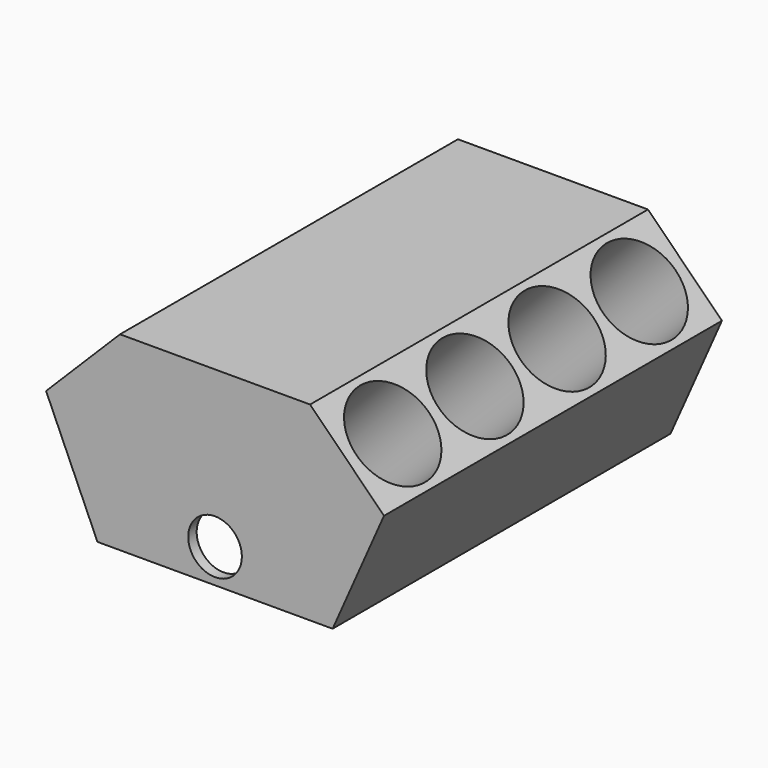
from build123d import *

# Parameters (mm, degrees)
F1_DEPTH  = 100
F2_R      = 21.59
F4_DEPTH  = 52
F3_R      = 21.59
F5_DEPTH  = 52
F6_DEPTH  = 2.5
F7_DEPTH  = 95
F8_DEPTH  = 2.5
F3_R_2    = 24
F9_DEPTH  = 51
F10_START = 43.5
F10_DEPTH = 5
F11_START = 43.5
F11_DEPTH = 5
F2_R_2    = 24
F12_DEPTH = 52


# Not quite as in the source:
# - a feature names something its author has since deleted; it is built from what else it names


with BuildPart() as f1:
    # F0 (on Front) → F1 (new body, symmetric)
    with BuildSketch(Plane.XZ):
        Polygon((-80, 0), (-55.6696653366, -55), (-51.7864015908, -55), (-51.7864015908, -38.9201976359), (-18.3995570987, -3.0922384467), (18.3995570987, -3.0922384467), (51.7864015908, -38.9201976359), (51.7864015908, -55), (55.6696653366, -55), (80, 0), (45, 35), (-45, 35), align=None)
        with BuildLine():
            Line((-18.3995570987, -3.0922384467), (-51.7864015908, -38.9201976359))
            Line((-51.7864015908, -38.9201976359), (-12.7, -38.9201976359))
            ThreePointArc((-12.7, -38.9201976359), (0, -26.2201976359), (12.7, -38.9201976359))
            Line((12.7, -38.9201976359), (51.7864015908, -38.9201976359))
            Line((51.7864015908, -38.9201976359), (18.3995570987, -3.0922384467))
            Line((18.3995570987, -3.0922384467), (-18.3995570987, -3.0922384467))
        make_face()
        with BuildLine():
            Line((-51.7864015908, -38.9201976359), (-51.7864015908, -55))
            Line((-51.7864015908, -55), (51.7864015908, -55))
            Line((51.7864015908, -55), (51.7864015908, -38.9201976359))
            Line((51.7864015908, -38.9201976359), (12.7, -38.9201976359))
            ThreePointArc((12.7, -38.9201976359), (0, -51.6201976359), (-12.7, -38.9201976359))
            Line((-12.7, -38.9201976359), (-51.7864015908, -38.9201976359))
        make_face()
    extrude(amount=F1_DEPTH, both=True)

    # F2 (on face) → F4 (cut)
    with BuildSketch(Plane(origin=(40, 0, 40), x_dir=(0, 1, 0), z_dir=(0.7071067812, 0, 0.7071067812))):
        with Locations((72.954, -31.8198008825)):
            Circle(F2_R)
        with Locations((24.318, -31.8198008825)):
            Circle(F2_R)
        with Locations((-24.318, -31.8198008824)):
            Circle(F2_R)
        with Locations((-72.954, -31.8198008825)):
            Circle(F2_R)
    extrude(amount=-F4_DEPTH, mode=Mode.SUBTRACT)

    # F3 (on face) → F5 (cut)
    with BuildSketch(Plane(origin=(-40, 0, 40), x_dir=(0, -1, 0), z_dir=(-0.7071067812, 0, 0.7071067812))):
        with Locations((-72.9539923101, -31.8285424949)):
            Circle(F3_R)
        with Locations((-24.3179954494, -31.8110678119)):
            Circle(F3_R)
        with Locations((24.3180014113, -31.8285424949)):
            Circle(F3_R)
        with Locations((72.9540014113, -31.8285424949)):
            Circle(F3_R)
    extrude(amount=-F5_DEPTH, mode=Mode.SUBTRACT)

    # F0 (on Front) → F6 (join, symmetric)
    with BuildSketch(Plane.XZ):
        with BuildLine():
            Line((-18.3995570987, -3.0922384467), (-51.7864015908, -38.9201976359))
            Line((-51.7864015908, -38.9201976359), (-12.7, -38.9201976359))
            ThreePointArc((-12.7, -38.9201976359), (0, -26.2201976359), (12.7, -38.9201976359))
            Line((12.7, -38.9201976359), (51.7864015908, -38.9201976359))
            Line((51.7864015908, -38.9201976359), (18.3995570987, -3.0922384467))
            Line((18.3995570987, -3.0922384467), (-18.3995570987, -3.0922384467))
        make_face()
    extrude(amount=F6_DEPTH, both=True)

    # F0 (on Front) → F7 (cut, symmetric)
    with BuildSketch(Plane.XZ):
        with BuildLine():
            Line((-18.3995570987, -3.0922384467), (-51.7864015908, -38.9201976359))
            Line((-51.7864015908, -38.9201976359), (-12.7, -38.9201976359))
            ThreePointArc((-12.7, -38.9201976359), (0, -26.2201976359), (12.7, -38.9201976359))
            Line((12.7, -38.9201976359), (51.7864015908, -38.9201976359))
            Line((51.7864015908, -38.9201976359), (18.3995570987, -3.0922384467))
            Line((18.3995570987, -3.0922384467), (-18.3995570987, -3.0922384467))
        make_face()
        with BuildLine():
            Line((-51.7864015908, -38.9201976359), (-51.7864015908, -55))
            Line((-51.7864015908, -55), (51.7864015908, -55))
            Line((51.7864015908, -55), (51.7864015908, -38.9201976359))
            Line((51.7864015908, -38.9201976359), (12.7, -38.9201976359))
            ThreePointArc((12.7, -38.9201976359), (0, -51.6201976359), (-12.7, -38.9201976359))
            Line((-12.7, -38.9201976359), (-51.7864015908, -38.9201976359))
        make_face()
    extrude(amount=F7_DEPTH, both=True, mode=Mode.SUBTRACT)

    # F0 (on Front) → F8 (join, symmetric)
    with BuildSketch(Plane.XZ):
        with BuildLine():
            Line((-18.3995570987, -3.0922384467), (-51.7864015908, -38.9201976359))
            Line((-51.7864015908, -38.9201976359), (-12.7, -38.9201976359))
            ThreePointArc((-12.7, -38.9201976359), (0, -26.2201976359), (12.7, -38.9201976359))
            Line((12.7, -38.9201976359), (51.7864015908, -38.9201976359))
            Line((51.7864015908, -38.9201976359), (18.3995570987, -3.0922384467))
            Line((18.3995570987, -3.0922384467), (-18.3995570987, -3.0922384467))
        make_face()
    extrude(amount=F8_DEPTH, both=True)



with BuildPart() as f9:
    # F3 (on face) → F9 (new body)
    with BuildSketch(Plane(origin=(-40, 0, 40), x_dir=(0, -1, 0), z_dir=(-0.7071067812, 0, 0.7071067812))):
        with Locations((24.3180014113, -31.8285424949)):
            Circle(F3_R_2)
        with Locations((24.3180014113, -31.8285424949)):
            Circle(F3_R, mode=Mode.SUBTRACT)
    extrude(amount=-F9_DEPTH)


with BuildPart() as f9b:
    # F3 (on face) → F9, piece 2 (new body)
    with BuildSketch(Plane(origin=(-40, 0, 40), x_dir=(0, -1, 0), z_dir=(-0.7071067812, 0, 0.7071067812))):
        with Locations((72.9540014113, -31.8285424949)):
            Circle(F3_R_2)
        with Locations((72.9540014113, -31.8285424949)):
            Circle(F3_R, mode=Mode.SUBTRACT)
    extrude(amount=-F9_DEPTH)


with BuildPart() as f9c:
    # F3 (on face) → F9, piece 3 (new body)
    with BuildSketch(Plane(origin=(-40, 0, 40), x_dir=(0, -1, 0), z_dir=(-0.7071067812, 0, 0.7071067812))):
        with Locations((-24.3180014113, -31.8285424949)):
            Circle(F3_R_2)
        with Locations((-24.3179954494, -31.8110678119)):
            Circle(F3_R, mode=Mode.SUBTRACT)
    extrude(amount=-F9_DEPTH)


with BuildPart() as f9d:
    # F3 (on face) → F9, piece 4 (new body)
    with BuildSketch(Plane(origin=(-40, 0, 40), x_dir=(0, -1, 0), z_dir=(-0.7071067812, 0, 0.7071067812))):
        with Locations((-72.9540014113, -31.8285424949)):
            Circle(F3_R_2)
        with Locations((-72.9539923101, -31.8285424949)):
            Circle(F3_R, mode=Mode.SUBTRACT)
    extrude(amount=-F9_DEPTH)


with BuildPart() as f1_1:
    add(f1.part)

    add(f9.part)  # F10 merges F9

    add(f9b.part)  # F10 merges F9b
    # F8_face (on face) → F10 (join)
    with BuildSketch(Plane(origin=(0, -2.5, -22.7617883235), x_dir=(1, 0, 0), z_dir=(0, -1, 0)).offset(F10_START)):
        with BuildLine():
            Line((-18.3995570987, 19.6695498768), (-51.7864015908, -16.1584093124))
            Line((-51.7864015908, -16.1584093124), (-12.7, -16.1584093124))
            ThreePointArc((-12.7, -16.1584093124), (0, -3.4584093124), (12.7, -16.1584093124))
            Line((12.7, -16.1584093124), (51.7864015908, -16.1584093124))
            Line((51.7864015908, -16.1584093124), (18.3995570987, 19.6695498768))
            Line((18.3995570987, 19.6695498768), (-18.3995570987, 19.6695498768))
        make_face()
    extrude(amount=F10_DEPTH)


    add(f9c.part)  # F11 merges F9c

    add(f9d.part)  # F11 merges F9d
    # F8_face1 (on face) → F11 (join)
    with BuildSketch(Plane(origin=(0, 2.5, -22.7617883235), x_dir=(1, 0, 0), z_dir=(0, 1, 0)).offset(F11_START)):
        with BuildLine():
            Line((-51.7864015908, 16.1584093124), (-18.3995570987, -19.6695498768))
            Line((-18.3995570987, -19.6695498768), (18.3995570987, -19.6695498768))
            Line((18.3995570987, -19.6695498768), (51.7864015908, 16.1584093124))
            Line((51.7864015908, 16.1584093124), (12.7, 16.1584093124))
            ThreePointArc((12.7, 16.1584093124), (0, 3.4584093124), (-12.7, 16.1584093124))
            Line((-12.7, 16.1584093124), (-51.7864015908, 16.1584093124))
        make_face()
    extrude(amount=F11_DEPTH)


with BuildPart() as f12:
    # F2 (on face) → F12 (new body)
    with BuildSketch(Plane(origin=(40, 0, 40), x_dir=(0, 1, 0), z_dir=(0.7071067812, 0, 0.7071067812))):
        with Locations((-72.954, -31.8198008825)):
            Circle(F2_R_2)
        with Locations((-72.954, -31.8198008825)):
            Circle(F2_R, mode=Mode.SUBTRACT)
    extrude(amount=-F12_DEPTH)


with BuildPart() as f12b:
    # F2 (on face) → F12, piece 2 (new body)
    with BuildSketch(Plane(origin=(40, 0, 40), x_dir=(0, 1, 0), z_dir=(0.7071067812, 0, 0.7071067812))):
        with Locations((-24.318, -31.8198008824)):
            Circle(F2_R_2)
        with Locations((-24.318, -31.8198008824)):
            Circle(F2_R, mode=Mode.SUBTRACT)
    extrude(amount=-F12_DEPTH)


with BuildPart() as f12c:
    # F2 (on face) → F12, piece 3 (new body)
    with BuildSketch(Plane(origin=(40, 0, 40), x_dir=(0, 1, 0), z_dir=(0.7071067812, 0, 0.7071067812))):
        with Locations((24.318, -31.8198008825)):
            Circle(F2_R_2)
        with Locations((24.318, -31.8198008825)):
            Circle(F2_R, mode=Mode.SUBTRACT)
    extrude(amount=-F12_DEPTH)


with BuildPart() as f12d:
    # F2 (on face) → F12, piece 4 (new body)
    with BuildSketch(Plane(origin=(40, 0, 40), x_dir=(0, 1, 0), z_dir=(0.7071067812, 0, 0.7071067812))):
        with Locations((72.954, -31.8198008825)):
            Circle(F2_R_2)
        with Locations((72.954, -31.8198008825)):
            Circle(F2_R, mode=Mode.SUBTRACT)
    extrude(amount=-F12_DEPTH)


with BuildPart() as f1_2:
    add(f1_1.part)

    # F13: union F12b, F12, F12d, F12c
    add(f12b.part)
    add(f12.part)
    add(f12d.part)
    add(f12c.part)


solid = f1_2.part
